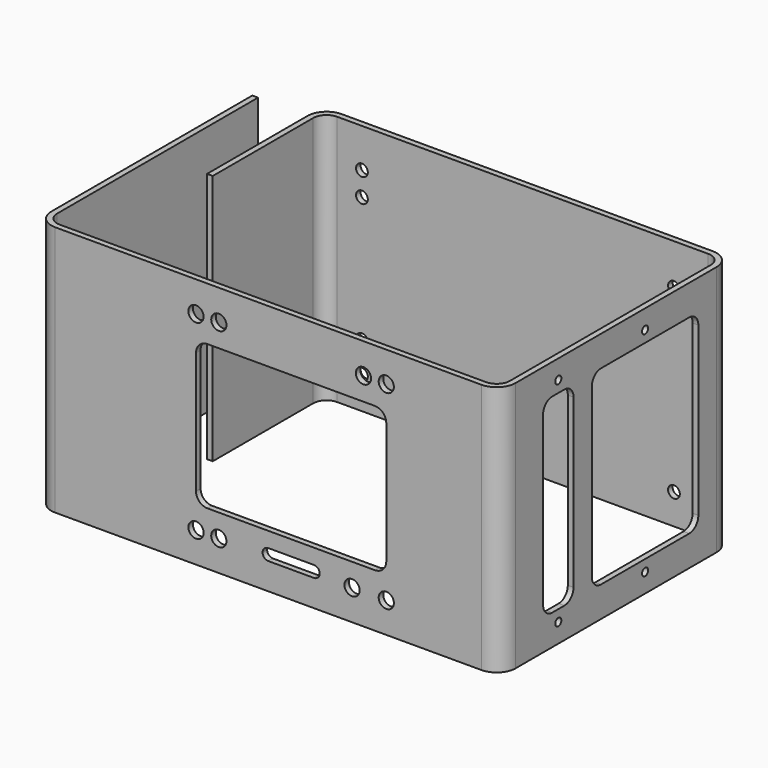
from build123d import *

# Parameters (mm, degrees)
F1_DEPTH = 66
F2_R     = 2
F3_DEPTH = 25
F4_R     = 1.55
F5_DEPTH = 25
F6_R     = 1
F7_DEPTH = 25


# Not quite as in the source:
# - a feature names something its author has since deleted; it is built from what else it names


with BuildPart() as f1:
    # F0 (on Top) → F1 (new body)
    with BuildSketch(Plane.XY):
        with BuildLine():
            Line((-66.75, -33), (-66.75, 33))
            Line((-66.75, 33), (-68.25, 33))
            Line((-68.25, 33), (-68.25, -33))
            ThreePointArc((-68.25, -33), (-66.7855339059, -36.5355339059), (-63.25, -38))
            Line((-63.25, -38), (48.75, -38))
            ThreePointArc((48.75, -38), (52.2855339059, -36.5355339059), (53.75, -33))
            Line((53.75, -33), (53.75, 33))
            ThreePointArc((53.75, 33), (52.2855339059, 36.5355339059), (48.75, 38))
            Line((48.75, 38), (-48.75, 38))
            ThreePointArc((-48.75, 38), (-52.2855339059, 36.5355339059), (-53.75, 33))
            Line((-53.75, 33), (-53.75, 0))
            Line((-53.75, 0), (-52.25, 0))
            Line((-52.25, 0), (-52.25, 33))
            ThreePointArc((-52.25, 33), (-51.2248737342, 35.4748737342), (-48.75, 36.5))
            Line((-48.75, 36.5), (48.75, 36.5))
            ThreePointArc((48.75, 36.5), (51.2248737342, 35.4748737342), (52.25, 33))
            Line((52.25, 33), (52.25, -33))
            ThreePointArc((52.25, -33), (51.2248737342, -35.4748737342), (48.75, -36.5))
            Line((48.75, -36.5), (-63.25, -36.5))
            ThreePointArc((-63.25, -36.5), (-65.7248737342, -35.4748737342), (-66.75, -33))
        make_face()
    extrude(amount=F1_DEPTH)

    # F2 (on face) → F3 (cut)
    with BuildSketch(Plane.XZ.offset(38)):
        with BuildLine():
            Line((20.75, 52), (-23.25, 52))
            ThreePointArc((-23.25, 52), (-25.3713203436, 51.1213203436), (-26.25, 49))
            Line((-26.25, 49), (-26.25, 17))
            ThreePointArc((-26.25, 17), (-25.3713203436, 14.8786796564), (-23.25, 14))
            Line((-23.25, 14), (20.75, 14))
            ThreePointArc((20.75, 14), (22.8713203436, 14.8786796564), (23.75, 17))
            Line((23.75, 17), (23.75, 49))
            ThreePointArc((23.75, 49), (22.8713203436, 51.1213203436), (20.75, 52))
        make_face()
        with Locations((-26.25, 58)):
            Circle(F2_R)
        with Locations((23.75, 58)):
            Circle(F2_R)
        with Locations((23.75, 8)):
            Circle(F2_R)
        with Locations((-26.25, 8)):
            Circle(F2_R)
        with BuildLine():
            ThreePointArc((-8.75, 8.5), (-8.3106601718, 7.4393398282), (-7.25, 7))
            Line((-7.25, 7), (4.75, 7))
            ThreePointArc((4.75, 7), (5.8106601718, 7.4393398282), (6.25, 8.5))
            ThreePointArc((6.25, 8.5), (5.8106601718, 9.5606601718), (4.75, 10))
            Line((4.75, 10), (-7.25, 10))
            ThreePointArc((-7.25, 10), (-8.3106601718, 9.5606601718), (-8.75, 8.5))
        make_face()
        with Locations((-20.25, 8)):
            Circle(F2_R)
        with Locations((-20.25, 58)):
            Circle(F2_R)
        with Locations((17.75, 58)):
            Circle(F2_R)
        with Locations((14.75, 8)):
            Circle(F2_R)
    extrude(amount=-F3_DEPTH, mode=Mode.SUBTRACT)

    # F4 (on face) → F5 (cut)
    with BuildSketch(Plane(origin=(0, 38, 0), x_dir=(-1, 0, 0), z_dir=(0, 1, 0))):
        with Locations((-39.74, 55.25)):
            Circle(F4_R)
        with Locations((-39.74, 8)):
            Circle(F4_R)
        with Locations((42.25, 8.5)):
            Circle(F4_R)
        with Locations((42.25, 55.75)):
            Circle(F4_R)
        with Locations((42.25, 16.5)):
            Circle(F4_R)
        with Locations((42.25, 49.5)):
            Circle(F4_R)
    extrude(amount=-F5_DEPTH, mode=Mode.SUBTRACT)

    # F6 (on face) → F7 (cut)
    with BuildSketch(Plane.YZ.offset(53.75)):
        with BuildLine():
            Line((-17, 58), (-21, 58))
            ThreePointArc((-21, 58), (-23.1213203436, 57.1213203436), (-24, 55))
            Line((-24, 55), (-24, 11))
            ThreePointArc((-24, 11), (-23.1213203436, 8.8786796564), (-21, 8))
            Line((-21, 8), (-17, 8))
            ThreePointArc((-17, 8), (-14.8786796564, 8.8786796564), (-14, 11))
            Line((-14, 11), (-14, 55))
            ThreePointArc((-14, 55), (-14.8786796564, 57.1213203436), (-17, 58))
        make_face()
        with BuildLine():
            Line((24, 58), (-5, 58))
            ThreePointArc((-5, 58), (-7.1213203436, 57.1213203436), (-8, 55))
            Line((-8, 55), (-8, 11))
            ThreePointArc((-8, 11), (-7.1213203436, 8.8786796564), (-5, 8))
            Line((-5, 8), (24, 8))
            ThreePointArc((24, 8), (26.1213203436, 8.8786796564), (27, 11))
            Line((27, 11), (27, 55))
            ThreePointArc((27, 55), (26.1213203436, 57.1213203436), (24, 58))
        make_face()
        with Locations((-19, 61)):
            Circle(F6_R)
        with Locations((9.5, 61)):
            Circle(F6_R)
        with Locations((9.5, 5)):
            Circle(F6_R)
        with Locations((-19, 5)):
            Circle(F6_R)
    extrude(amount=-F7_DEPTH, mode=Mode.SUBTRACT)


solid = f1.part
